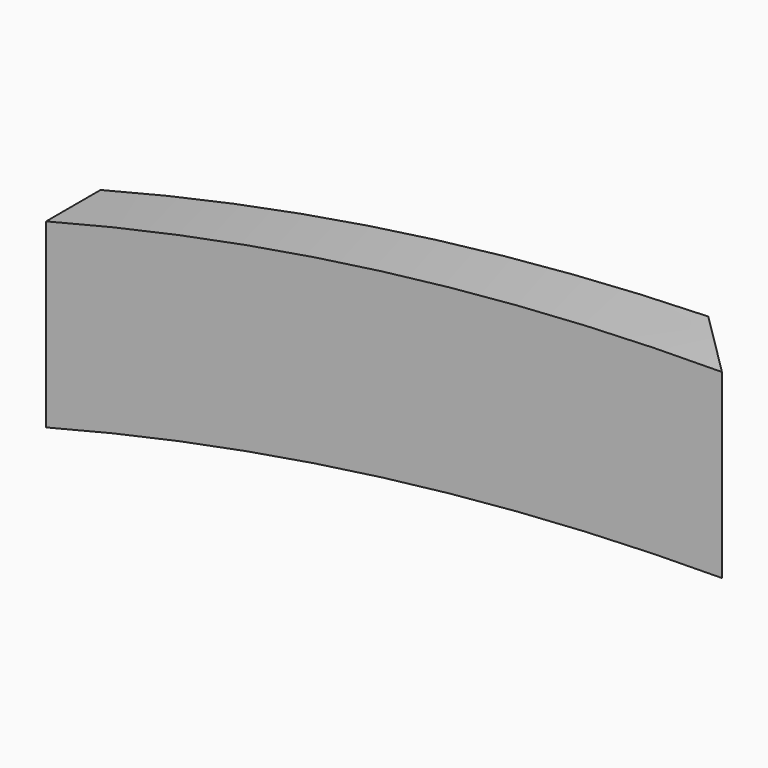
from build123d import *

# Parameters (mm, degrees)
F1_DEPTH    = 7.5
F2_T1_DEPTH = 61.1469278075


# Not quite as in the source:
# - a fillet or chamfer that OpenCascade refuses, or shapes differently, is made with other operations: its cross-section is extruded or revolved along the edge and cut away or added
# - a feature names something its author has since deleted; it is built from what else it names


with BuildPart() as f1:
    # F0 (on Front) → F1 (new body)
    with BuildSketch(Plane.XZ):
        with BuildLine():
            Line((-75.013438644, 20), (-75.013438644, 0))
            ThreePointArc((-75.013438644, 0), (-37.8148015278, 7.2106165672), (0, 9.613194347))
            Line((0, 9.613194347), (0, 29.613194347))
            ThreePointArc((0, 29.613194347), (-37.8148015278, 27.2106165672), (-75.013438644, 20))
        make_face()
    extrude(amount=F1_DEPTH)

    # F2: chamfer of 8 on 1 edges, made by hand

    # F2_s2 → F2_t1 (cut)
    with BuildSketch(Plane.XY.offset(-10.9602695567)):
        Polygon((0, -8), (-8, 0), (0, 0), align=None)
    extrude(amount=F2_T1_DEPTH, mode=Mode.SUBTRACT)


solid = f1.part
